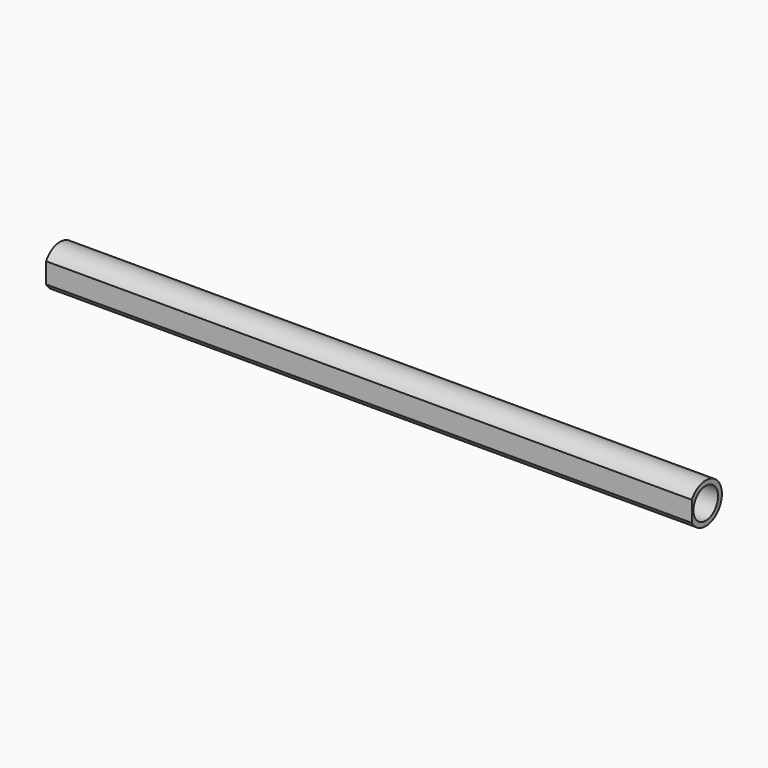
from build123d import *

# Parameters (mm, degrees)
F0_R     = 12.7
F1_DEPTH = 533.4


# Not quite as in the source:
# - a feature names something its author has since deleted; it is built from what else it names


with BuildPart() as f1:
    # F0 (on Right) → F1 (new body)
    with BuildSketch(Plane.YZ):
        with BuildLine():
            ThreePointArc((-14.431408661, -8.4048286305), (4.352870312, -16.1232509221), (16.7005, 0))
            ThreePointArc((16.7005, 0), (4.352870312, 16.1232509221), (-14.431408661, 8.4048286305))
            Line((-14.431408661, 8.4048286305), (-14.431408661, -8.4048286305))
        make_face()
        Circle(F0_R, mode=Mode.SUBTRACT)
    extrude(amount=F1_DEPTH)


solid = f1.part
